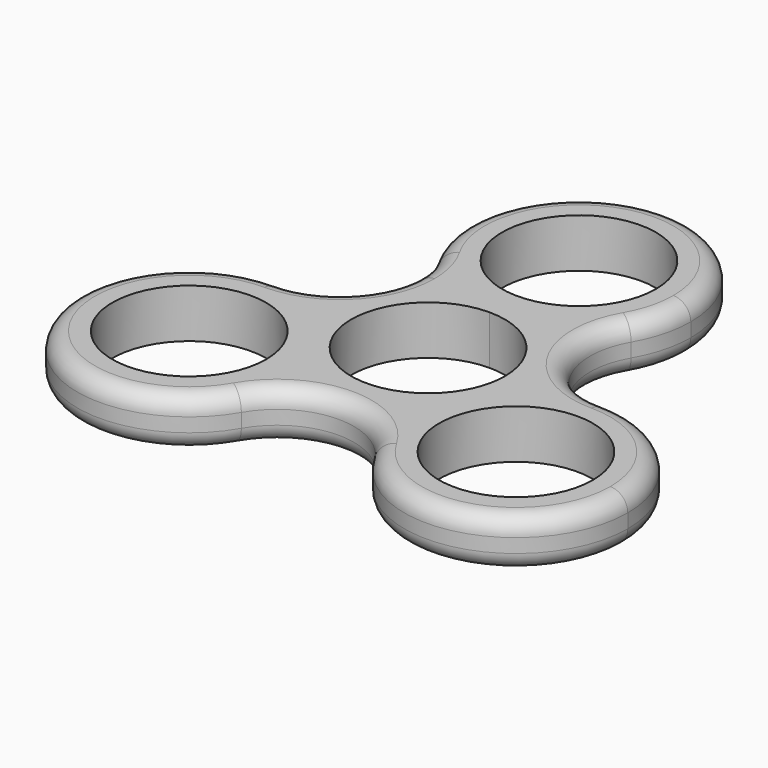
from build123d import *

# Parameters (mm, degrees)
F0_R     = 11
F1_DEPTH = 7
F2_R     = 2.5


with BuildPart() as f1:
    # F0 (on Top) → F1 (new body)
    with BuildSketch(Plane.XY):
        with BuildLine():
            ThreePointArc((-13.8564063169, 18.9999997511), (-7.9999998612, 13.1435934593), (3.3e-08, 11))
            ThreePointArc((3.3e-08, 11), (8.0000000671, 13.1435935782), (13.8564065215, 19.0000001056))
            ThreePointArc((13.8564065215, 19.0000001056), (15.4548132364, 22.8588953372), (16, 27))
            ThreePointArc((16, 27), (-4.1411048604, 42.4548131834), (-13.8564063169, 18.9999997511))
        make_face()
        with Locations((0, 27)):
            Circle(F0_R, mode=Mode.SUBTRACT)
        with BuildLine():
            ThreePointArc((-9.5262794581, -5.4999999715), (-9.5262794251, 5.5000000286), (3.3e-08, 11))
            ThreePointArc((3.3e-08, 11), (-7.9999998612, 13.1435934593), (-13.8564063169, 18.9999997511))
            ThreePointArc((-13.8564063169, 18.9999997511), (-12.7575017758, 16.3470093573), (-12.3826859022, 13.5))
            ThreePointArc((-12.3826859022, 13.5), (-15.6045113091, 5.7218254069), (-23.3826859022, 2.5))
            ThreePointArc((-23.3826859022, 2.5), (-15.3826859164, 0.3564064688), (-9.5262794581, -5.4999999715))
        make_face()
        with BuildLine():
            ThreePointArc((9.5262794719, -21.5000000524), (7.3826859022, -13.5000000639), (9.5262794079, -5.5000000584))
            ThreePointArc((9.5262794079, -5.5000000584), (-5.02e-08, -11), (-9.5262794581, -5.4999999715))
            ThreePointArc((-9.5262794581, -5.4999999715), (-7.9278726858, -9.3588952624), (-7.3826859022, -13.5))
            ThreePointArc((-7.3826859022, -13.5), (-7.9278726602, -17.641104642), (-9.5262793592, -21.4999998571))
            ThreePointArc((-9.5262793592, -21.4999998571), (1.127e-07, -16), (9.5262794719, -21.5000000524))
        make_face()
        with BuildLine():
            ThreePointArc((3.3e-08, 11), (7.7781746047, 7.7781745814), (11, 0))
            ThreePointArc((11, 0), (10.6251840805, -2.8470095287), (9.5262794079, -5.5000000584))
            ThreePointArc((9.5262794079, -5.5000000584), (15.382685873, 0.3564064437), (23.3826859022, 2.5))
            ThreePointArc((23.3826859022, 2.5), (13.8564064301, 8.0000000528), (13.8564065215, 19.0000001056))
            ThreePointArc((13.8564065215, 19.0000001056), (8.0000000671, 13.1435935782), (3.3e-08, 11))
        make_face()
        with BuildLine():
            ThreePointArc((-7.3826859022, -13.5), (-7.9278726858, -9.3588952624), (-9.5262794581, -5.4999999715))
            ThreePointArc((-9.5262794581, -5.4999999715), (-15.3826859164, 0.3564064688), (-23.3826859022, 2.5))
            ThreePointArc((-23.3826859022, 2.5), (-37.2390923215, -21.5000000714), (-9.5262793592, -21.4999998571))
            ThreePointArc((-9.5262793592, -21.4999998571), (-7.9278726602, -17.641104642), (-7.3826859022, -13.5))
        make_face()
        with Locations((-23.3826859022, -13.5)):
            Circle(F0_R, mode=Mode.SUBTRACT)
        with BuildLine():
            ThreePointArc((23.3826859022, 2.5), (15.382685873, 0.3564064437), (9.5262794079, -5.5000000584))
            ThreePointArc((9.5262794079, -5.5000000584), (7.3826859022, -13.5000000639), (9.5262794719, -21.5000000524))
            ThreePointArc((9.5262794719, -21.5000000524), (27.523790653, -28.9548132128), (39.3826859022, -13.5))
            ThreePointArc((39.3826859022, -13.5), (34.6963944012, -2.186291501), (23.3826859022, 2.5))
        make_face()
        with Locations((23.3826859022, -13.5)):
            Circle(F0_R, mode=Mode.SUBTRACT)
    extrude(amount=F1_DEPTH)

    # F2
    f2_edges = [f1.edges().sort_by_distance(p)[0] for p in [
        (0, 43, 7),
        (0, 43, 0),
        (13.856406, 8, 7),
        (13.856406, 8, 0),
        (37.239092, -21.5, 0),
        (37.239092, -21.5, 7),
        (0, -16, 7),
        (0, -16, 0),
        (-37.239092, -21.5, 0),
        (-37.239092, -21.5, 7),
        (-13.856407, 8, 7),
        (-13.856407, 8, 0),
    ]]
    fillet(f2_edges, radius=F2_R)


solid = f1.part
